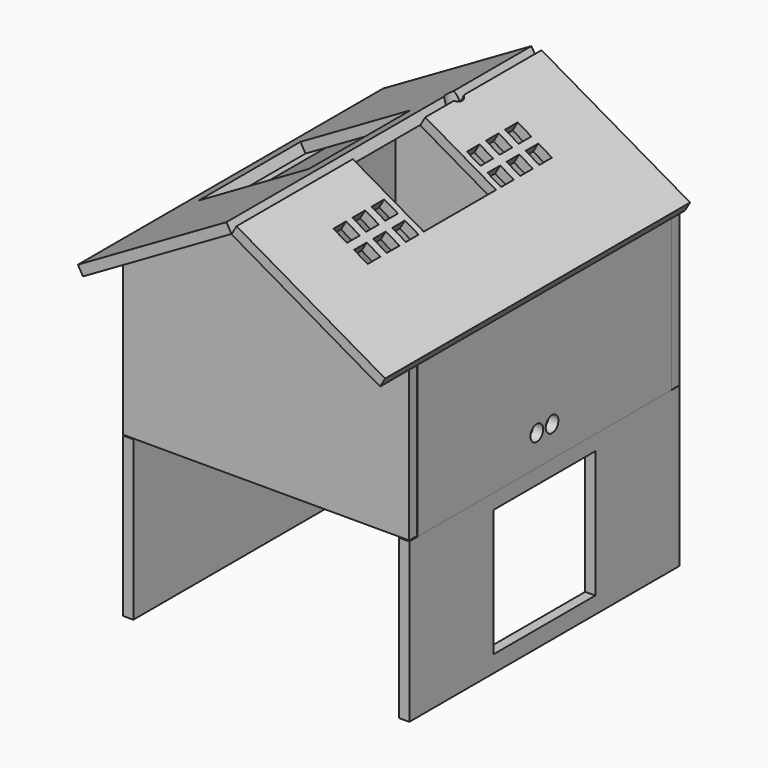
from build123d import *

# Parameters (mm, degrees)
F1_DEPTH       = 3.175
F2_W           = 3.175
F2_H           = 50
F3_DEPTH       = 100
F4_W           = 3.175
F4_H           = 50
F5_DEPTH       = 100
F7_DEPTH       = 3.175
F8_W           = 83.65
F8_H           = 3.175
F9_DEPTH       = 100
F10_W          = 3.175
F10_H          = 50
F11_DEPTH      = 103.175
F11_DEPTH_BACK = 3.175
F12_W          = 40
F12_H          = 40
F13_DEPTH      = 25
F15_DEPTH      = 120
F18_DEPTH      = 120
F19_W          = 40
F19_H          = 40
F20_DEPTH      = 25
F21_R          = 2.5
F22_DEPTH      = 3.175
F23_W          = 5
F23_H          = 5
F23_W_2        = 25.7498108172
F23_H_2        = 28.499999997
F24_DEPTH      = 3.175
F25_R          = 2.5
F26_DEPTH      = 53.8262042049
F27_W          = 40
F27_H          = 40
F28_DEPTH      = 25
F29_W          = 3.175
F29_H          = 106.35
F30_DEPTH      = 50
F31_R          = 2.5
F32_DEPTH      = 25


# Not quite as in the source:
# - a length typed as a fraction of an inch, garbled in the dataset ("3 / 203.2 mm" for 3/8 in), is restored


with BuildPart() as f1:
    # F0 (on Front) → F1 (new body)
    with BuildSketch(Plane.XZ):
        Polygon((-45, 25), (-45, -25), (45, -25), (45, 25), (0, 25), align=None)
        Polygon((0, 50.9807621135), (-45, 25), (0, 25), align=None)
        Polygon((0, 25), (45, 25), (0, 50.9807621135), align=None)
    extrude(amount=-F1_DEPTH)


with BuildPart() as f3:
    # F2 (on Front) → F3 (new body)
    with BuildSketch(Plane.XZ):
        with Locations((43.454606086, -0.0529892971)):
            Rectangle(F2_W, F2_H)
    extrude(amount=F3_DEPTH)

    # F21 (on face) → F22 (cut, through all)
    with BuildSketch(Plane.YZ.offset(45.042106086)):
        with Locations((-53, -15.3529893)):
            Circle(F21_R)
        with Locations((-47, -15.3529893)):
            Circle(F21_R)
    extrude(amount=-F22_DEPTH, mode=Mode.SUBTRACT)


with BuildPart() as f5:
    # F4 (on Front) → F5 (new body)
    with BuildSketch(Plane.XZ):
        with Locations((-43.4125, 0)):
            Rectangle(F4_W, F4_H)
    extrude(amount=F5_DEPTH)

    # F31 (on face) → F32 (cut)
    with BuildSketch(Plane(origin=(-45, 0, 0), x_dir=(0, -1, 0), z_dir=(-1, 0, 0))):
        with Locations((50, -15.05299)):
            Circle(F31_R)
    extrude(amount=-F32_DEPTH, mode=Mode.SUBTRACT)


with BuildPart() as f7:
    # F6 (on face) → F7 (new body)
    with BuildSketch(Plane.XZ.offset(100)):
        Polygon((-1.9791e-06, 51.2161863094), (-45.0000019791, 25.2354241958), (-1.9791e-06, 25.2354241958), align=None)
        Polygon((-1.9791e-06, 25.2354241958), (-45.0000019791, 25.2354241958), (-45.0000019791, -24.7645758042), (44.9999980209, -24.7645758042), (44.9999980209, 25.2354241958), align=None)
        Polygon((-1.9791e-06, 51.2161863094), (-1.9791e-06, 25.2354241958), (44.9999980209, 25.2354241958), align=None)
    extrude(amount=F7_DEPTH)


with BuildPart() as f9:
    # F8 (on Front) → F9 (new body)
    with BuildSketch(Plane.XZ):
        with Locations((0, -23.4125)):
            Rectangle(F8_W, F8_H)
    extrude(amount=F9_DEPTH)

    # F12 (on Top) → F13 (cut, through all)
    with BuildSketch(Plane.XY):
        with Locations((0, -50)):
            Rectangle(F12_W, F12_H)
    extrude(amount=-F13_DEPTH, mode=Mode.SUBTRACT)


with BuildPart() as f11:
    # F10 (on Front) → F11 (new body, two sides)
    with BuildSketch(Plane.XZ) as f11_sk:
        with Locations((43.454606086, -50.0529892971)):
            Rectangle(F10_W, F10_H)
    extrude(amount=F11_DEPTH)
    extrude(f11_sk.sketch, amount=-F11_DEPTH_BACK)

    # F27 (on face) → F28 (cut)
    with BuildSketch(Plane(origin=(41.867106086, 0, 0), x_dir=(0, -1, 0), z_dir=(-1, 0, 0))):
        with Locations((49.995, -49.7845411301)):
            Rectangle(F27_W, F27_H)
    extrude(amount=-F28_DEPTH, mode=Mode.SUBTRACT)


with BuildPart() as f15:
    # F14 (on face) → F15 (new body)
    with BuildSketch(Plane(origin=(0, 3.175, 0), x_dir=(-1, 0, 0), z_dir=(0, 1, 0))):
        Polygon((1.5875, 53.8252042049), (0, 51.0755735479), (46.7653718044, 24.0755735479), (48.3528718044, 26.8252042049), align=None)
    extrude(amount=-F15_DEPTH)

    # F19 (on face) → F20 (cut)
    with BuildSketch(Plane(origin=(-23.7038721027, 0, 41.0563108179), x_dir=(0.8660254038, 0, 0.5), z_dir=(-0.5, 0, 0.8660254038))):
        with Locations((-1.4622132261, -56.825)):
            Rectangle(F19_W, F19_H)
    extrude(amount=-F20_DEPTH, mode=Mode.SUBTRACT)


with BuildPart() as f18:
    # F17 (on face) → F18 (new body)
    with BuildSketch(Plane(origin=(0, 3.175, 0), x_dir=(-1, 0, 0), z_dir=(0, 1, 0))):
        Polygon((-48.3528718044, 26.7303927705), (-46.7653718044, 23.9807621135), (-45, 25), (0, 50.9807621135), (-1.5875, 53.7303927705), align=None)
    extrude(amount=-F18_DEPTH)

    # F23 (on face) → F24 (cut, through all)
    with BuildSketch(Plane(origin=(23.6628175473, 0, 40.9852022422), x_dir=(0.8660254038, 0, -0.5), z_dir=(0.5, 0, 0.8660254038))):
        with Locations((-9.7399080962, -90.575)):
            Rectangle(F23_W, F23_H)
        with Locations((-9.7400026881, -83.0750000006)):
            Rectangle(F23_W, F23_H)
        with Locations((-9.74009728, -75.5750000012)):
            Rectangle(F23_W, F23_H)
        with Locations((-9.7405702396, -38.0750000042)):
            Rectangle(F23_W, F23_H)
        with Locations((-9.7406648315, -30.5750000048)):
            Rectangle(F23_W, F23_H)
        with Locations((-9.7407594235, -23.0750000054)):
            Rectangle(F23_W, F23_H)
        with Locations((-2.2399080962, -90.575)):
            Rectangle(F23_W, F23_H)
        with Locations((-2.2400026881, -83.0750000006)):
            Rectangle(F23_W, F23_H)
        with Locations((-2.24009728, -75.5750000012)):
            Rectangle(F23_W, F23_H)
        with Locations((-2.2405702396, -38.0750000042)):
            Rectangle(F23_W, F23_H)
        with Locations((-2.2406648315, -30.5750000048)):
            Rectangle(F23_W, F23_H)
        with Locations((-2.2407594235, -23.0750000054)):
            Rectangle(F23_W, F23_H)
        with Locations((-12.6154756482, -56.8250000027)):
            Rectangle(F23_W_2, F23_H_2)
    extrude(amount=-F24_DEPTH, mode=Mode.SUBTRACT)


with BuildPart() as f26_tool:
    # F25 (on Top) → F26 (new body, through all)
    with BuildSketch(Plane.XY):
        with Locations((0.0346281956, -29.325)):
            Circle(F25_R)
    extrude(amount=F26_DEPTH)


with BuildPart() as f15_1:
    add(f15.part)

    # F26: cut by f26_tool
    add(f26_tool.part, mode=Mode.SUBTRACT)


with BuildPart() as f18_1:
    add(f18.part)

    # F26: cut by f26_tool
    add(f26_tool.part, mode=Mode.SUBTRACT)


with BuildPart() as f30:
    # F29 (on face) → F30 (new body)
    with BuildSketch(Plane(origin=(0, 0, -25), x_dir=(1, 0, 0), z_dir=(0, 0, -1))):
        with Locations((-43.4125, 50)):
            Rectangle(F29_W, F29_H)
    extrude(amount=F30_DEPTH)


solid = Compound([f1.part, f3.part, f5.part, f7.part, f9.part, f11.part, f15_1.part, f18_1.part, f30.part])
